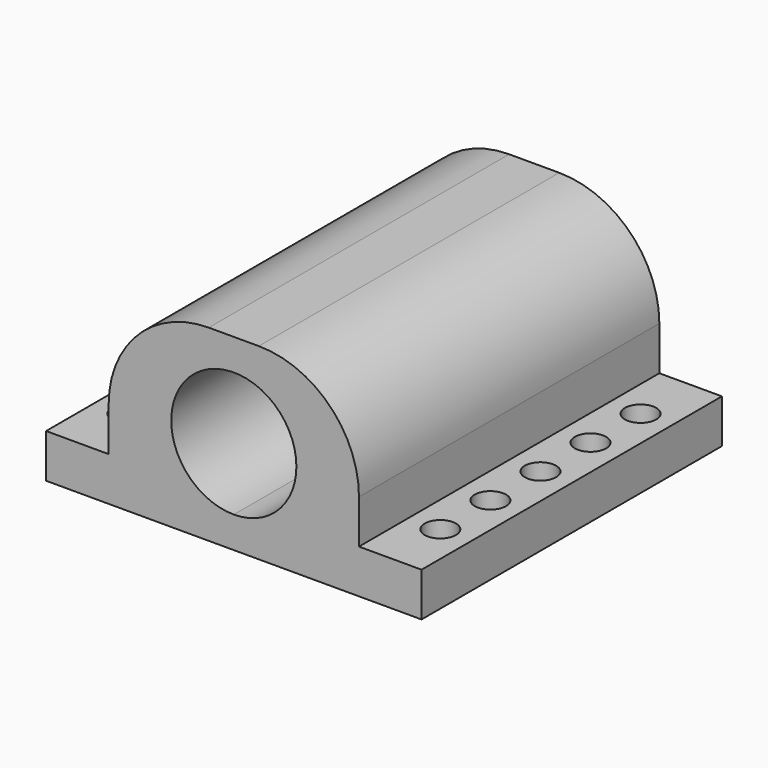
from build123d import *

# Parameters (mm, degrees)
F0_W     = 25.4
F0_H     = 38.1
F1_DEPTH = 19.05
F3_DEPTH = 38.1
F4_R     = 10.16
F5_W     = 38.1
F5_H     = 4.445
F6_DEPTH = 6.35
F9_D     = 3.175


# Not quite as in the source:
# - a pattern or mirror of a feature is missing from the dataset's text; its kind, count and spacing are read off the source's solid


with BuildPart() as f1:
    # F0 (on Top) → F1 (new body)
    with BuildSketch(Plane.XY):
        with Locations((12.7, 19.05)):
            Rectangle(F0_W, F0_H)
    extrude(amount=F1_DEPTH)

    # F2 (on face) → F3 (cut, through all)
    with BuildSketch(Plane.XZ):
        with BuildLine():
            ThreePointArc((19.05, 9.525), (8.2098719395, 14.0151280605), (12.7, 3.175))
            ThreePointArc((12.7, 3.175), (17.1901280605, 5.0348719395), (19.05, 9.525))
        make_face()
    extrude(amount=-F3_DEPTH, mode=Mode.SUBTRACT)

    # F4
    f4_edges = [f1.edges().sort_by_distance(p)[0] for p in [
        (25.4, 19.05, 19.05),
        (0, 19.05, 19.05),
    ]]
    fillet(f4_edges, radius=F4_R)

    # F5 (on face) → F6 (join)
    with BuildSketch(Plane.YZ.offset(25.4)):
        with Locations((19.05, 2.2225)):
            Rectangle(F5_W, F5_H)
    f6 = extrude(amount=F6_DEPTH)

    # F6_copies: F6 across plane
    add(f6.mirror(Plane(origin=(12.7, 0, 0), x_dir=(0, 0, -1), z_dir=(-1, 0, 0))))

    # F9 (through all)
    with Locations(Plane.XY.offset(4.445)):
        with Locations((28.575, 6.35), (28.575, 12.7), (28.575, 19.05), (28.575, 25.4), (28.575, 31.75)):
            f9 = Hole(F9_D / 2)

    # F9_copies: F9 across plane
    add(f9.mirror(Plane(origin=(12.7, 0, 0), x_dir=(0, 0, -1), z_dir=(-1, 0, 0))), mode=Mode.SUBTRACT)


solid = f1.part
